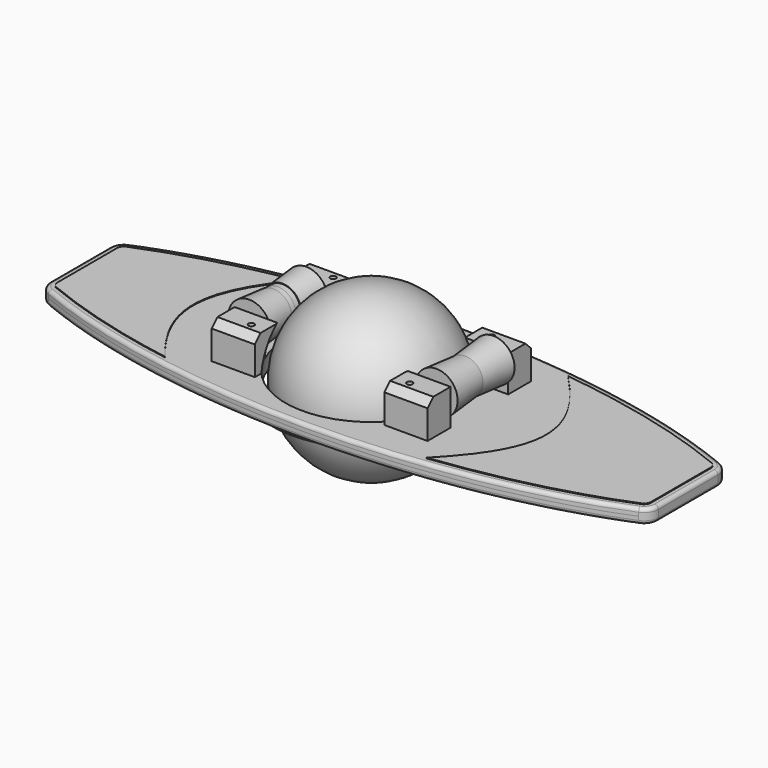
from build123d import *

# Parameters (mm, degrees)
F1_DEPTH       = 10
F1_DEPTH_BACK  = 10
F5_DEPTH       = 50
F10_R          = 6
F11_DEPTH      = 20
F12_W          = 30
F12_H          = 50
F13_DEPTH      = 92.1819621658
F9_R           = 25
F9_R_2         = 6
F14_DEPTH      = 49.5
F14_TAPER      = -5
F14_DEPTH_BACK = 49.5
F14_TAPER_BACK = -5
F15_R          = 6
F16_DEPTH      = 99
F18_R          = 4
F19_DEPTH      = 172.501
F20_SIZE       = 10
F25_R          = 5
F27_R          = 29.3306888445
F27_R_2        = 25
F28_DEPTH      = 8
F28_DEPTH_BACK = 8
F29_R          = 6
F30_DEPTH      = 140
F32_R          = 4
F33_DEPTH      = 122.501
F34_R          = 137.582607431
F34_R_2        = 4
F34_R_3        = 122.582607431
F35_DEPTH      = 3
F36_R          = 6
F37_DEPTH      = 20
F38_R          = 2.5
F39_DEPTH      = 25
F41_DEPTH      = 2
F43_DEPTH      = 2
F44_DEPTH      = 3


# Not quite as in the source:
# - ends of sketch curves that miss each other by under 0.0002 mm in the source are joined
# - the dataset's text gives a spline's control points without its knots; the knots are read off the source's solid
# - a feature names something its author has since deleted; it is built from what else it names


with BuildPart() as f1:
    # F0 (on Top) → F1 (new body, two sides)
    with BuildSketch(Plane.XY) as f1_sk:
        with BuildLine():
            ThreePointArc((-392.6284171425, 70.2464264801), (-401.6217980804, 62.8811582507), (-405, 51.7583965174))
            Line((-405, 51.7583965174), (-405, -51.7583965174))
            ThreePointArc((-405, -51.7583965174), (-401.6217980804, -62.8811582507), (-392.6284171425, -70.2464264801))
            add(Edge.make_bspline(
                [(-392.6284171425, -70.2464264801), (-161.7777589352, -165.4986043478), (191.9310719644, -166.8238805218), (427.5856115688, -70.2271477332)],
                knots=[14.7166958992, 14.7166958992, 14.7166958992, 14.7166958992, 830.5440792194, 830.5440792194, 830.5440792194, 830.5440792194], degree=3))
            ThreePointArc((427.5856115688, -70.2271477332), (436.6089167524, -62.8635009826), (440, -51.7215135336))
            Line((440, -51.7215135336), (440, 51.7215135336))
            ThreePointArc((440, 51.7215135336), (436.6089167524, 62.8635009826), (427.5856115688, 70.2271477332))
            add(Edge.make_bspline(
                [(-392.6284171425, 70.2464264801), (-161.7777589352, 165.4986043478), (191.9310719644, 166.8238805218), (427.5856115688, 70.2271477332)],
                knots=[14.7166958992, 14.7166958992, 14.7166958992, 14.7166958992, 830.5440792194, 830.5440792194, 830.5440792194, 830.5440792194], degree=3))
        make_face()
    extrude(amount=F1_DEPTH)
    extrude(f1_sk.sketch, amount=-F1_DEPTH_BACK)


with BuildPart() as f5:
    # F4 (on face) → F5 (new body)
    with BuildSketch(Plane.XY.offset(10)):
        with BuildLine():
            Line((180, -50), (109.0871211464, -50))
            ThreePointArc((109.0871211464, -50), (100.6211059783, -65.3864896727), (90, -79.3725393319))
            Line((90, -79.3725393319), (90, -90))
            Line((90, -90), (180, -90))
            Line((180, -90), (180, -50))
        make_face()
        with BuildLine():
            ThreePointArc((90, -79.3725393319), (100.6211059783, -65.3864896727), (109.0871211464, -50))
            Line((109.0871211464, -50), (90, -50))
            Line((90, -50), (90, -79.3725393319))
        make_face()
    extrude(amount=F5_DEPTH)


with BuildPart() as f6_tool:
    # F3 (on Front) → F6 (revolve)
    with BuildSketch(Plane.XZ):
        with BuildLine():
            Line((0, 120), (0, -120))
            ThreePointArc((0, -120), (120, 0), (0, 120))
        make_face()
    revolve(axis=Axis((0, 0, 7.9277970081), (0, 0, -1)))


with BuildPart() as f1_1:
    add(f1.part)

    # F6: cut by f6_tool
    add(f6_tool.part, mode=Mode.SUBTRACT)


with BuildPart() as f5_1:
    add(f5.part)

    # F6: cut by f6_tool
    add(f6_tool.part, mode=Mode.SUBTRACT)

    # F10 (on face) → F11 (cut)
    with BuildSketch(Plane(origin=(0, -50, 0), x_dir=(-1, 0, 0), z_dir=(0, 1, 0))):
        with Locations((-130, 46)):
            Circle(F10_R)
    extrude(amount=-F11_DEPTH, mode=Mode.SUBTRACT)

    # F12 (on face) → F13 (cut, through all)
    with BuildSketch(Plane(origin=(0, -50, 0), x_dir=(-1, 0, 0), z_dir=(0, 1, 0))):
        with Locations((-165, 35)):
            Rectangle(F12_W, F12_H)
    extrude(amount=-F13_DEPTH, mode=Mode.SUBTRACT)


with BuildPart() as f8:
    # F7 (on Front) → F8 (revolve)
    with BuildSketch(Plane.XZ):
        with BuildLine():
            Line((0, 112.5), (0, -112.5))
            ThreePointArc((0, -112.5), (112.5, 0), (0, 112.5))
        make_face()
    revolve(axis=Axis((0, 0, -14.2883807421), (0, 0, -1)))


with BuildPart() as f14:
    # F9 (on Front) → F14 (new body, two sides)
    with BuildSketch(Plane.XZ) as f14_sk:
        with Locations((130, 46)):
            Circle(F9_R)
        with Locations((130, 46)):
            Circle(F9_R_2, mode=Mode.SUBTRACT)
    extrude(amount=F14_DEPTH, taper=F14_TAPER)
    extrude(f14_sk.sketch, amount=-F14_DEPTH_BACK, taper=F14_TAPER_BACK)

    # F15 (on face) → F16 (cut, through all)
    with BuildSketch(Plane(origin=(0, 49.5, 0), x_dir=(-1, 0, 0), z_dir=(0, 1, 0))):
        with Locations((-130, 46)):
            Circle(F15_R)
    extrude(amount=-F16_DEPTH, mode=Mode.SUBTRACT)


with BuildPart() as f19_tool:
    # F18 (on face) → F19 (new body, through all)
    with BuildSketch(Plane.XY.offset(60)):
        with Locations((110, -70.9807621135)):
            Circle(F18_R)
    extrude(amount=-F19_DEPTH)


with BuildPart() as f1_2:
    add(f1_1.part)

    # F19: cut by f19_tool
    add(f19_tool.part, mode=Mode.SUBTRACT)

    # F25
    f25_edges = [f1_2.edges().sort_by_distance(p)[0] for p in [
        (17.467205, 142.18093, 10),
        (17.467205, 142.18093, -10),
        (436.608917, 62.863501, 10),
        (436.608917, 62.863501, -10),
        (-401.621798, 62.881158, 10),
        (-401.621798, 62.881158, -10),
        (440, 0, 10),
        (-405, 0, 10),
        (436.608917, -62.863501, 10),
        (-401.621798, -62.881158, 10),
        (15.677142, -142.180129, 10),
        (440, 0, -10),
        (-405, 0, -10),
        (436.608917, -62.863501, -10),
        (-401.621798, -62.881158, -10),
        (15.677142, -142.180129, -10),
    ]]
    fillet(f25_edges, radius=F25_R)

    # F32 (on face) → F33 (cut, through all)
    with BuildSketch(Plane(origin=(0, 0, -10), x_dir=(1, 0, 0), z_dir=(0, 0, -1))):
        with Locations((110, 70.9807621135)):
            Circle(F32_R)
        with Locations((-110, 70.9807621135)):
            Circle(F32_R)
        with Locations((-110, -70.9807621135)):
            Circle(F32_R)
        with Locations((110, -70.9807621135)):
            Circle(F32_R)
    extrude(amount=-F33_DEPTH, mode=Mode.SUBTRACT)

    # F40 (on face) → F41 (cut)
    with BuildSketch(Plane.XY.offset(10)):
        with BuildLine():
            ThreePointArc((-388.8142106349, 61.0024165), (-393.3109035367, 57.3197803929), (-395.0000054103, 51.7583965174))
            Line((-395.0000054103, 51.7583965174), (-395.0000054103, -51.7583965174))
            ThreePointArc((-395.0000054103, -51.7583965174), (-393.3109035367, -57.3197803929), (-388.8142106349, -61.0024165))
            add(Edge.make_bspline(
                [(-388.8142106349, -61.0024165), (-380.7599654306, -64.325709588), (-364.5420161063, -70.660883818), (-339.9149663155, -79.3104623444), (-319.1627133582, -85.8615046963), (-302.4327515499, -90.7346010773), (-291.9247849534, -93.6317369077), (-283.4886671286, -95.8627911164), (-275.2199334803, -97.9888623984), (-269.0552155141, -99.5092394536), (-265, -100.4823495192)],
                knots=[0, 0, 0, 0, 0.0262647482, 0.0525294963, 0.0787942445, 0.0919266185, 0.1050589926, 0.1116251796, 0.1181913667, 0.1307949048, 0.1307949048, 0.1307949048, 0.1307949048], degree=3))
            Line((-265, -100.4823495192), (-265, 100.4826562863))
            add(Edge.make_bspline(
                [(-265, 100.4826562863), (-273.4862317212, 98.4462531292), (-298.6661082767, 92.0513051627), (-340.1349823153, 79.6679674281), (-372.6954578935, 67.6532370567), (-388.8142106349, 61.0024165)],
                knots=[0.7088381862, 0.7088381862, 0.7088381862, 0.7088381862, 0.7354105324, 0.7879398561, 0.8404691799, 0.8404691799, 0.8404691799, 0.8404691799], degree=3))
        make_face()
        with BuildLine():
            add(Edge.make_bspline(
                [(-194.999999747, 114.7615431629), (-210.0933750499, 112.1951754969), (-233.4985221479, 107.7264101621), (-256.7102944357, 102.4718999385), (-265, 100.4826562863)],
                knots=[0.6363873264, 0.6363873264, 0.6363873264, 0.6363873264, 0.6828812086, 0.7088381862, 0.7088381862, 0.7088381862, 0.7088381862], degree=3))
            Line((-265, 100.4826562863), (-265, -100.4823495192))
            add(Edge.make_bspline(
                [(-265, -100.4823495192), (-264.8298458845, -100.5231805631), (-260.4342269802, -101.576747768), (-251.8083593497, -103.5821309241), (-234.8791094797, -107.2915834913), (-215.9472479094, -111.0729729561), (-201.2299952894, -113.7020839465), (-194.999999952, -114.7614743203)],
                knots=[0.1307949048, 0.1307949048, 0.1307949048, 0.1307949048, 0.1313237408, 0.1444561148, 0.1575884889, 0.1838532371, 0.203110561, 0.203110561, 0.203110561, 0.203110561], degree=3))
            add(Edge.make_bspline(
                [(-194.999999747, 114.7615431629), (-265, 30), (-265, -30), (-194.999999952, -114.7614743203)],
                knots=[0, 0, 0, 0, 229.5230192534, 229.5230192534, 229.5230192534, 229.5230192534], degree=3))
        make_face()
    extrude(amount=-F41_DEPTH, mode=Mode.SUBTRACT)

    # F42 (on face) → F43 (cut)
    with BuildSketch(Plane.XY.offset(10)):
        with BuildLine():
            add(Edge.make_bspline(
                [(423.7928057844, 60.9743306334), (415.7301798765, 64.2792672653), (399.4989352483, 70.5857370911), (374.8597591702, 79.2093474731), (354.102157905, 85.7489443375), (337.3701181012, 90.6172165981), (326.8615253256, 93.5128958948), (318.4255371739, 95.7434925005), (309.9871189481, 97.9133042046), (299.4292130857, 100.515136035), (286.7462800679, 103.4661292778), (269.8177574006, 107.1798705762), (248.6251026008, 111.4202179304), (223.145742627, 115.8999358461), (198.6032654036, 119.6488990024), (182.5434406721, 121.7679346131), (175.0000000076, 122.692021673)],
                knots=[0, 0, 0, 0, 0.0262646619, 0.0525293237, 0.0787939856, 0.0919263165, 0.1050586475, 0.111624813, 0.1181909784, 0.1313233094, 0.1444556403, 0.1575879712, 0.1838526331, 0.210117295, 0.2363819568, 0.2596148406, 0.2596148406, 0.2596148406, 0.2596148406], degree=3))
            add(Edge.make_bspline(
                [(175, 122.6920216108), (265, 30), (265, -30), (175, -122.6920365428)],
                knots=[0, 0, 0, 0, 245.3840581535, 245.3840581535, 245.3840581535, 245.3840581535], degree=3))
            add(Edge.make_bspline(
                [(175.0000000002, -122.6920365442), (178.4976346638, -122.2635810342), (186.2984733727, -121.2737774788), (202.6748476097, -119.0335211176), (232.6349660904, -114.4334985836), (275.0876283164, -106.4355840386), (325.4246593025, -94.3702780571), (375.0819970522, -79.5595551888), (407.6602924303, -67.5871804614), (423.7928057844, -60.9743306334)],
                knots=[0.5803028052, 0.5803028052, 0.5803028052, 0.5803028052, 0.5909568334, 0.6040892075, 0.6303539557, 0.682883452, 0.7354129483, 0.7879424446, 0.8404719409, 0.8404719409, 0.8404719409, 0.8404719409], degree=3))
            ThreePointArc((423.7928057844, -60.9743306334), (428.3044583762, -57.2925072581), (430, -51.7215135336))
            Line((430, -51.7215135336), (430, 51.7215135336))
            ThreePointArc((430, 51.7215135336), (428.3044583762, 57.2925072581), (423.7928057844, 60.9743306334))
        make_face()
    extrude(amount=-F43_DEPTH, mode=Mode.SUBTRACT)


with BuildPart() as f5_2:
    add(f5_1.part)

    # F19: cut by f19_tool
    add(f19_tool.part, mode=Mode.SUBTRACT)

    # F20
    f20_edges = [f5_2.edges().sort_by_distance(p)[0] for p in [
        (120, -90, 60),
    ]]
    chamfer(f20_edges, length=F20_SIZE)


with BuildPart() as f21_1:
    # F21: instance of F5
    add(f5_2.part.mirror(Plane.XZ))


with BuildPart() as f22_1:
    # F22: instance of F5
    add(f5_2.part.mirror(Plane.YZ))


with BuildPart() as f22_2:
    # F22: instance of F14
    add(f14.part.mirror(Plane.YZ))

    # F27 (on Front) → F28 (cut, two sides)
    with BuildSketch(Plane.XZ) as f28_sk:
        with Locations((-130, 46)):
            Circle(F27_R)
        with Locations((-130, 46)):
            Circle(F27_R_2, mode=Mode.SUBTRACT)
    extrude(amount=-F28_DEPTH, mode=Mode.SUBTRACT)
    extrude(f28_sk.sketch, amount=F28_DEPTH_BACK, mode=Mode.SUBTRACT)


with BuildPart() as f22_3:
    # F22: instance of F21_1
    add(f21_1.part.mirror(Plane.YZ))


with BuildPart() as f30:
    # F29 (on face) → F30 (new body, through all)
    with BuildSketch(Plane.XZ.offset(-70)):
        with Locations((130, 46)):
            Circle(F29_R)
    extrude(amount=F30_DEPTH)


with BuildPart() as f31_1:
    # F31: instance of F30
    add(f30.part.mirror(Plane.YZ))

    # F36 (on face) → F37 (cut)
    with BuildSketch(Plane.XZ.offset(70)):
        with Locations((-130, 46)):
            Circle(F36_R)
    extrude(amount=-F37_DEPTH, mode=Mode.SUBTRACT)

    # F38 (on face) → F39 (cut)
    with BuildSketch(Plane.XZ.offset(50)):
        with Locations((-130, 46)):
            Circle(F38_R)
    extrude(amount=-F39_DEPTH, mode=Mode.SUBTRACT)


with BuildPart() as f35:
    # F34 (on face) → F35 (new body)
    with BuildSketch(Plane(origin=(0, 0, -10), x_dir=(1, 0, 0), z_dir=(0, 0, -1))):
        Circle(F34_R)
        with Locations((-110, -70.9807621135)):
            Circle(F34_R_2, mode=Mode.SUBTRACT)
        with Locations((110, -70.9807621135)):
            Circle(F34_R_2, mode=Mode.SUBTRACT)
        with Locations((-110, 70.9807621135)):
            Circle(F34_R_2, mode=Mode.SUBTRACT)
        Circle(F34_R_3, mode=Mode.SUBTRACT)
        with Locations((110, 70.9807621135)):
            Circle(F34_R_2, mode=Mode.SUBTRACT)
    extrude(amount=F35_DEPTH)


with BuildPart() as f44:
    # F44 (new): a face of the model
    f44_faces = [f1_2.part.faces().sort_by_distance(p)[0] for p in [
        (-303.7721961555, 0.0001398775, 8),
    ]]
    extrude(f44_faces, amount=F44_DEPTH)


with BuildPart() as f44b:
    # F44#2 (new): a face of the model
    f44_2_faces = [f1_2.part.faces().sort_by_distance(p)[0] for p in [
        (312.749799276, -9.54125e-05, 8),
    ]]
    extrude(f44_2_faces, amount=F44_DEPTH)


solid = Compound([f8.part, f14.part, f1_2.part, f5_2.part, f21_1.part, f22_1.part, f22_2.part, f22_3.part, f30.part, f31_1.part, f35.part, f44.part, f44b.part])
